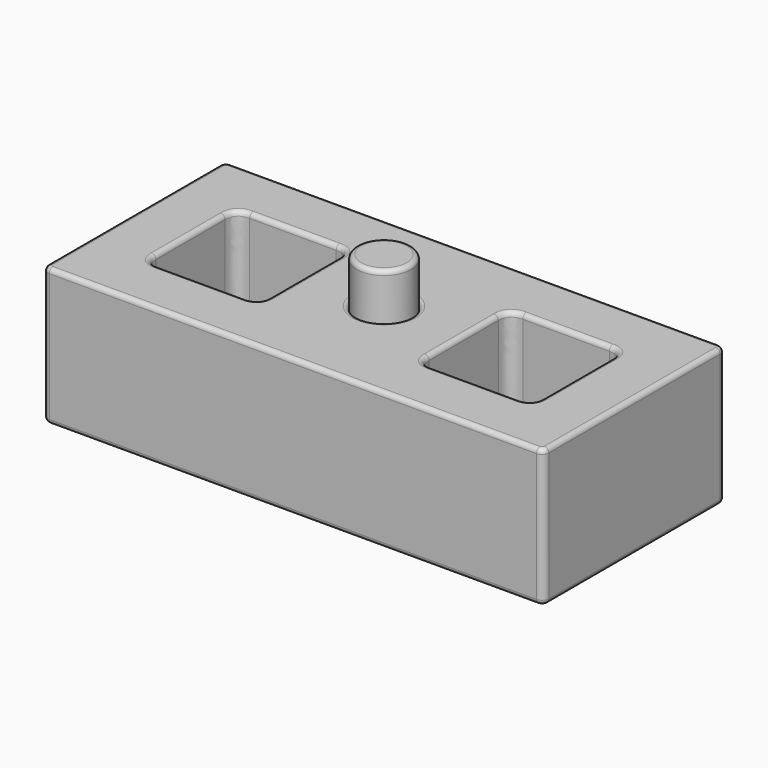
from build123d import *

# Parameters (mm, degrees)
F0_R        = 6
F1_DEPTH    = 10
F0_W        = 110
F0_H        = 50
F0_W_2      = 25
F0_H_2      = 25
F2_DEPTH    = 30.17
F3_SIZE     = 5
F4_T1_DEPTH = 30.17
F5_R        = 1.5
F6_R        = 1
F6_2_R      = 1
F7_R        = 1
F8_R        = 1


# Not quite as in the source:
# - a fillet or chamfer that OpenCascade refuses, or shapes differently, is made with other operations: its cross-section is extruded or revolved along the edge and cut away or added


with BuildPart() as f1:
    # F0 (on Top) → F1 (new body, symmetric)
    with BuildSketch(Plane.XY):
        Circle(F0_R)
    extrude(amount=F1_DEPTH, both=True)

    # F6
    f6_edges = [f1.edges().sort_by_distance(p)[0] for p in [
        (-6, 0, 10),
    ]]
    fillet(f6_edges, radius=F6_R)


with BuildPart() as f2:
    # F0 (on Top) → F2 (new body)
    with BuildSketch(Plane.XY):
        Rectangle(F0_W, F0_H)
        with Locations((-30, 0)):
            Rectangle(F0_W_2, F0_H_2, mode=Mode.SUBTRACT)
        Circle(F0_R, mode=Mode.SUBTRACT)
        with Locations((30, 0)):
            Rectangle(F0_W_2, F0_H_2, mode=Mode.SUBTRACT)
    extrude(amount=-F2_DEPTH)

    # F3
    f3_edges = [f2.edges().sort_by_distance(p)[0] for p in [
        (-6, 0, -30.17),
    ]]
    chamfer(f3_edges, length=F3_SIZE)

    # F4: fillet of radius 3 on 8 edges, made by hand

    # F4_s2 → F4_t1 (join)
    with BuildSketch(Plane.XY.offset(-30.17)):
        with BuildLine():
            add(Edge.make_bspline(
                [(-42.5, 9.5), (-42.5, 12.5), (-39.5, 12.5)],
                knots=[0, 0, 0, 1, 1, 1], degree=2, weights=[1, 1, 1]))
            Line((-39.5, 12.5), (-42.5, 12.5))
            Line((-42.5, 12.5), (-42.5, 9.5))
        make_face()
        with BuildLine():
            add(Edge.make_bspline(
                [(-20.5, 12.5), (-17.5, 12.5), (-17.5, 9.5)],
                knots=[0, 0, 0, 1, 1, 1], degree=2, weights=[1, 1, 1]))
            Line((-17.5, 9.5), (-17.5, 12.5))
            Line((-17.5, 12.5), (-20.5, 12.5))
        make_face()
        with BuildLine():
            add(Edge.make_bspline(
                [(-17.5, -9.5), (-17.5, -12.5), (-20.5, -12.5)],
                knots=[0, 0, 0, 1, 1, 1], degree=2, weights=[1, 1, 1]))
            Line((-20.5, -12.5), (-17.5, -12.5))
            Line((-17.5, -12.5), (-17.5, -9.5))
        make_face()
        with BuildLine():
            add(Edge.make_bspline(
                [(-42.5, -9.5), (-42.5, -12.5), (-39.5, -12.5)],
                knots=[0, 0, 0, 1, 1, 1], degree=2, weights=[1, 1, 1]))
            Line((-39.5, -12.5), (-42.5, -12.5))
            Line((-42.5, -12.5), (-42.5, -9.5))
        make_face()
        with BuildLine():
            add(Edge.make_bspline(
                [(17.5, -9.5), (17.5, -12.5), (20.5, -12.5)],
                knots=[0, 0, 0, 1, 1, 1], degree=2, weights=[1, 1, 1]))
            Line((20.5, -12.5), (17.5, -12.5))
            Line((17.5, -12.5), (17.5, -9.5))
        make_face()
        with BuildLine():
            add(Edge.make_bspline(
                [(42.5, -9.5), (42.5, -12.5), (39.5, -12.5)],
                knots=[0, 0, 0, 1, 1, 1], degree=2, weights=[1, 1, 1]))
            Line((39.5, -12.5), (42.5, -12.5))
            Line((42.5, -12.5), (42.5, -9.5))
        make_face()
        with BuildLine():
            add(Edge.make_bspline(
                [(39.5, 12.5), (42.5, 12.5), (42.5, 9.5)],
                knots=[0, 0, 0, 1, 1, 1], degree=2, weights=[1, 1, 1]))
            Line((42.5, 9.5), (42.5, 12.5))
            Line((42.5, 12.5), (39.5, 12.5))
        make_face()
        with BuildLine():
            add(Edge.make_bspline(
                [(17.5, 9.5), (17.5, 12.5), (20.5, 12.5)],
                knots=[0, 0, 0, 1, 1, 1], degree=2, weights=[1, 1, 1]))
            Line((20.5, 12.5), (17.5, 12.5))
            Line((17.5, 12.5), (17.5, 9.5))
        make_face()
    extrude(amount=F4_T1_DEPTH)

    # F5
    f5_edges = [f2.edges().sort_by_distance(p)[0] for p in [
        (55, 25, -15.085),
        (55, -25, -15.085),
        (-55, 25, -15.085),
        (-55, -25, -15.085),
    ]]
    fillet(f5_edges, radius=F5_R)

    # F6#2
    f6_2_edges = [f2.edges().sort_by_distance(p)[0] for p in [
        (55, 0, 0),
        (54.56066, -24.56066, 0),
        (54.56066, 24.56066, 0),
        (0, -25, 0),
        (0, 25, 0),
        (-54.56066, -24.56066, 0),
        (-54.56066, 24.56066, 0),
        (-55, 0, 0),
        (-42.5, 0, 0),
        (-41.750012, 11.749988, 0),
        (-30, 12.5, 0),
        (-18.250012, 11.750012, 0),
        (-17.5, 0, 0),
        (-18.249988, -11.749988, 0),
        (-30, -12.5, 0),
        (-41.750012, -11.749988, 0),
        (-6, 0, 0),
        (17.5, 0, 0),
        (18.249988, 11.749988, 0),
        (30, 12.5, 0),
        (41.749988, 11.750012, 0),
        (42.5, 0, 0),
        (41.750012, -11.749988, 0),
        (30, -12.5, 0),
        (18.249988, -11.749988, 0),
    ]]
    fillet(f6_2_edges, radius=F6_2_R)

    # F7
    f7_edges = [f2.edges().sort_by_distance(p)[0] for p in [
        (0, -25, -30.17),
        (55, 0, -30.17),
        (0, 25, -30.17),
        (-55, 0, -30.17),
    ]]
    fillet(f7_edges, radius=F7_R)

    # F8
    f8_edges = [f2.edges().sort_by_distance(p)[0] for p in [
        (-17.5, 0, -30.17),
        (-30, 12.5, -30.17),
        (-42.5, 0, -30.17),
        (-30, -12.5, -30.17),
        (17.5, 0, -30.17),
        (30, 12.5, -30.17),
        (42.5, 0, -30.17),
        (30, -12.5, -30.17),
        (18.249988, 11.749988, -30.17),
        (41.749988, 11.750012, -30.17),
        (41.750012, -11.749988, -30.17),
        (18.249988, -11.749988, -30.17),
        (-18.249988, -11.749988, -30.17),
        (-18.250012, 11.750012, -30.17),
        (-41.750012, 11.749988, -30.17),
        (-41.750012, -11.749988, -30.17),
    ]]
    fillet(f8_edges, radius=F8_R)


solid = Compound([f1.part, f2.part])
